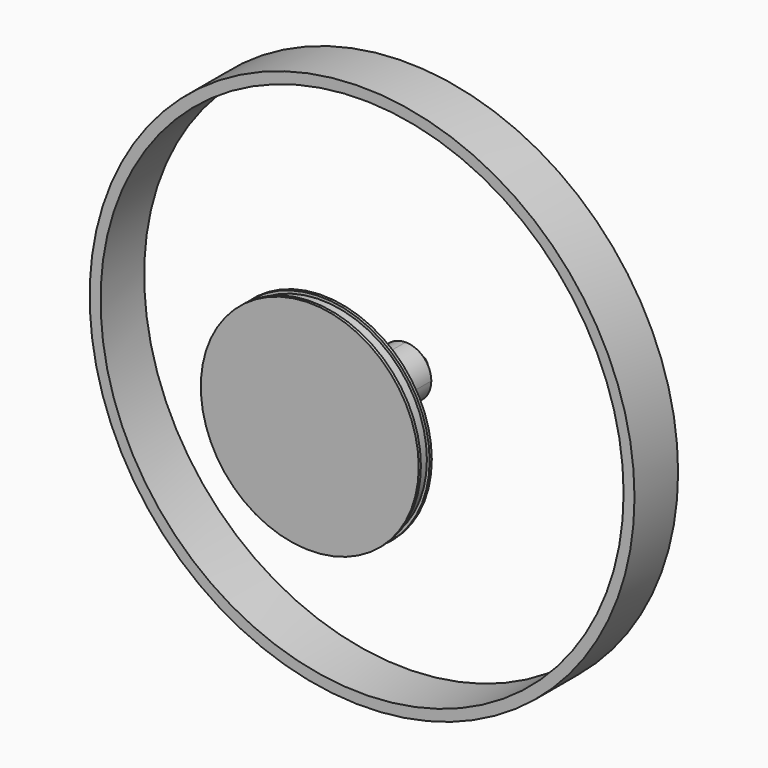
from build123d import *

# Parameters (mm, degrees)
F0_R          = 63.5
F1_DEPTH      = 6.35
F2_R          = 60.96
F3_DEPTH      = 12.701
F5_DEPTH      = 6.35
F6_R          = 2.170991
F7_DEPTH      = 17.78
F7_DEPTH_BACK = 10.16
F8_R          = 25.4
F9_DEPTH      = 0.635
F10_R         = 24.765
F11_DEPTH     = 2.54
F13_R         = 25.4
F14_DEPTH     = 0.635


# Not quite as in the source:
# - the program builds the solid bodies; features that only make, move or delete a surface that nothing else refers to are left out


with BuildPart() as f1:
    # F0 (on Front) → F1 (new body, symmetric)
    with BuildSketch(Plane.XZ):
        Circle(F0_R)
    extrude(amount=F1_DEPTH, both=True)

    # F2 (on face) → F3 (cut, through all)
    with BuildSketch(Plane.XZ.offset(6.35)):
        Circle(F2_R)
    extrude(amount=-F3_DEPTH, mode=Mode.SUBTRACT)


with BuildPart() as f5:
    # F4 (on Front) → F5 (new body, symmetric)
    with BuildSketch(Plane.XZ):
        with BuildLine():
            ThreePointArc((0, -5.980991), (4.229199, -4.229199), (5.980991, 0))
            ThreePointArc((5.980991, 0), (4.229199, 4.229199), (0, 5.980991))
            ThreePointArc((0, 5.980991), (-5.980991, 0), (0, -5.980991))
        make_face()
    extrude(amount=F5_DEPTH, both=True)

    # F6 (on Front) → F7 (join, two sides)
    with BuildSketch(Plane.XZ) as f7_sk:
        Circle(F6_R)
    extrude(amount=F7_DEPTH)
    extrude(f7_sk.sketch, amount=-F7_DEPTH_BACK)

    # F8 (on face) → F9 (join)
    with BuildSketch(Plane.XZ.offset(17.78)):
        Circle(F8_R)
    extrude(amount=F9_DEPTH)

    # F10 (on face) → F11 (join)
    with BuildSketch(Plane.XZ.offset(18.415)):
        Circle(F10_R)
    extrude(amount=F11_DEPTH)

    # F13 (on face) → F14 (join)
    with BuildSketch(Plane.XZ.offset(20.955)):
        Circle(F13_R)
    extrude(amount=F14_DEPTH)


solid = Compound([f1.part, f5.part])
